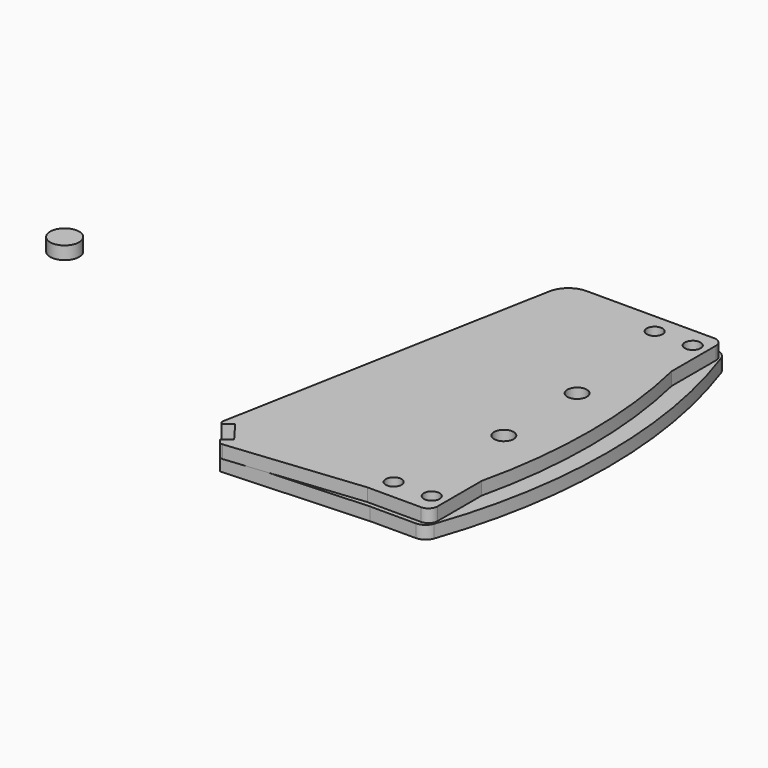
from build123d import *

# Parameters (mm, degrees)
F0_R     = 8.7
F0_R_2   = 10.75
F1_DEPTH = 14.2875
F2_R     = 8.7
F2_R_2   = 10.75
F3_DEPTH = 14.2875
F0_R_3   = 16
F4_DEPTH = 14.2875


# Not quite as in the source:
# - a length typed as a fraction of an inch, garbled in the dataset ("3 / 203.2 mm" for 3/8 in), is restored
# - a feature names something its author has since deleted; it is built from what else it names


with BuildPart() as f1:
    # F0 (on Top) → F1 (new body)
    with BuildSketch(Plane.XY):
        with BuildLine():
            Line((348.2189872385, -217.2652141408), (495.7062776099, -202))
            Line((495.7062776099, -202), (555, -202))
            ThreePointArc((555, -202), (562.0710678119, -199.0710678119), (565, -192))
            Line((565, -192), (565, -131.0534242208))
            ThreePointArc((565, -131.0534242208), (580, 0), (565, 131.0534242208))
            Line((565, 131.0534242208), (565, 192))
            ThreePointArc((565, 192), (562.0710678119, 199.0710678119), (555, 202))
            Line((555, 202), (414.1631860812, 202))
            ThreePointArc((414.1631860812, 202), (398.1915832415, 196.2329899582), (389.5886519187, 181.5926322185))
            Line((389.5886519187, 181.5926322185), (321.4556631787, -182.977483508))
            ThreePointArc((321.4556631787, -182.977483508), (321.501996532, -185.0348656396), (322.3730600039, -186.8993270748))
            Line((322.3730600039, -186.8993270748), (323.410873951, -188.2806902374))
            Line((323.410873951, -188.2806902374), (333.0048979686, -181.0727291422))
            Line((333.0048979686, -181.0727291422), (350.4241372821, -204.2582871847))
            Line((350.4241372821, -204.2582871847), (340.8301132645, -211.4662482799))
            Line((340.8301132645, -211.4662482799), (343.7067176257, -215.2950995966))
            ThreePointArc((343.7067176257, -215.2950995966), (345.7035463941, -216.8740607913), (348.2189872385, -217.2652141408))
        make_face()
        with Locations((507, -180)):
            Circle(F0_R, mode=Mode.SUBTRACT)
        with Locations((549, -180)):
            Circle(F0_R, mode=Mode.SUBTRACT)
        with Locations((527, -53.020531197)):
            Circle(F0_R_2, mode=Mode.SUBTRACT)
        with Locations((527, 47.979468803)):
            Circle(F0_R_2, mode=Mode.SUBTRACT)
        with Locations((507, 180)):
            Circle(F0_R, mode=Mode.SUBTRACT)
        with Locations((549, 180)):
            Circle(F0_R, mode=Mode.SUBTRACT)
    extrude(amount=F1_DEPTH)

    # F2 (on face) → F3 (join)
    with BuildSketch(Plane(origin=(0, 0, 0), x_dir=(1, 0, 0), z_dir=(0, 0, -1))):
        with BuildLine():
            Line((416.0266704213, -207), (553.0775391075, -207))
            ThreePointArc((553.0775391075, -207), (560.9475314042, -204.4911597734), (565.9135130702, -197.8903958685))
            ThreePointArc((565.9135130702, -197.8903958685), (599.5153985116, 0), (565.9135130702, 197.8903958685))
            ThreePointArc((565.9135130702, 197.8903958685), (560.9475314042, 204.4911597734), (553.0775391075, 207))
            Line((553.0775391075, 207), (502.4613982964, 207))
            Line((502.4613982964, 207), (343.7067176257, 215.2950995966))
            Line((343.7067176257, 215.2950995966), (340.8301132645, 211.4662482799))
            Line((340.8301132645, 211.4662482799), (350.4241372821, 204.2582871847))
            Line((350.4241372821, 204.2582871847), (333.0048979686, 181.0727291422))
            Line((333.0048979686, 181.0727291422), (323.410873951, 188.2806902374))
            Line((323.410873951, 188.2806902374), (321.4556631787, 182.977483508))
            Line((321.4556631787, 182.977483508), (324.5568533725, 166.3834475094))
            Line((324.5568533725, 166.3834475094), (400.2244110781, 131.3875502719))
            ThreePointArc((400.2244110781, 131.3875502719), (404.4521498311, 127.6974775298), (406.0266704213, 122.3112639511))
            Line((406.0266704213, 122.3112639511), (406.0266704213, -197))
            ThreePointArc((406.0266704213, -197), (408.9556026095, -204.0710678119), (416.0266704213, -207))
        make_face()
        with Locations((507, -180)):
            Circle(F2_R, mode=Mode.SUBTRACT)
        with Locations((549, -180)):
            Circle(F2_R, mode=Mode.SUBTRACT)
        with Locations((527, -47.979468803)):
            Circle(F2_R_2, mode=Mode.SUBTRACT)
        with Locations((527, 53.020531197)):
            Circle(F2_R_2, mode=Mode.SUBTRACT)
        with Locations((507, 180)):
            Circle(F2_R, mode=Mode.SUBTRACT)
        with Locations((549, 180)):
            Circle(F2_R, mode=Mode.SUBTRACT)
    extrude(amount=F3_DEPTH)


with BuildPart() as f4:
    # F0 (on Top) → F4 (new body)
    with BuildSketch(Plane.XY):
        Circle(F0_R_3)
    extrude(amount=F4_DEPTH)


solid = Compound([f1.part, f4.part])
